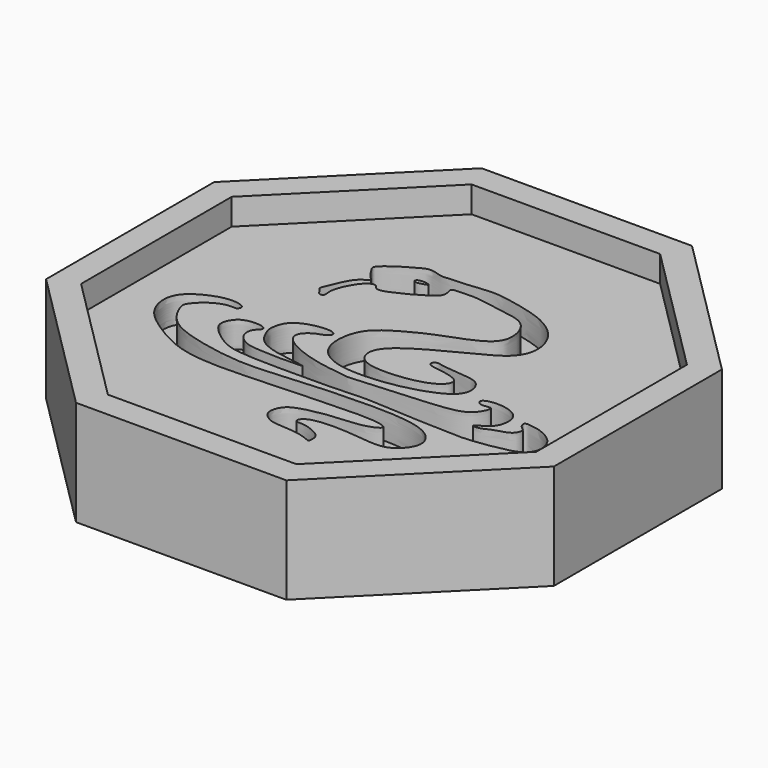
from build123d import *

# Parameters (mm, degrees)
F1_DEPTH = 25.4
F3_DEPTH = 6.35
F5_DEPTH = 6.35


with BuildPart() as f1:
    # F0 (on Top) → F1 (new body)
    with BuildSketch(Plane.XY):
        Polygon((-61.3372846899, 25.3607087968), (-61.3047391097, -25.4392807779), (-25.3607087968, -61.3372846899), (25.4392807779, -61.3047391097), (61.3372846899, -25.3607087968), (61.3047391097, 25.4392807779), (25.3607087968, 61.3372846899), (-25.4392807779, 61.3047391097), align=None)
    extrude(amount=F1_DEPTH)

    # F2 (on face) → F3 (cut)
    with BuildSketch(Plane.XY.offset(25.4)):
        Polygon((-54.9856008905, 22.734521413), (-54.9564255154, -22.8049569991), (-22.734521413, -54.9856008905), (22.8049569991, -54.9564255154), (54.9856008905, -22.734521413), (54.9564255154, 22.8049569991), (22.734521413, 54.9856008905), (-22.8049569991, 54.9564255154), align=None)
    extrude(amount=-F3_DEPTH, mode=Mode.SUBTRACT)

    # F4 (on face) → F5 (cut)
    with BuildSketch(Plane.XY.offset(19.05)):
        with BuildLine():
            add(Edge.make_bspline(
                [(0, 32.4928350747), (-2.02665443, 32.4515584663), (-6.1821896181, 31.7497065716), (-9.3396897547, 31.9242783794), (-11.5003480916, 31.3913149272), (-14.4774634916, 32.8444451189), (-17.4734169272, 31.4267092211), (-24.3950179391, 27.1323443805), (-23.4189738768, 25.4150859361), (-21.7980747865, 22.8958449868), (-20.2814454001, 21.9562019156), (-23.4921452503, 21.1361770855), (-25.5825772036, 15.5301374946), (-26.6320070635, 13.378526896), (-25.6067459699, 12.798784515), (-25.1286460968, 11.4356624756), (-23.5210478416, 11.6468537322), (-24.6057192979, 14.0162008911), (-21.7647301762, 20.1265801161), (-18.9984353167, 21.4468623697), (-18.2021783197, 20.2606055269), (-16.9086613099, 19.2202016185), (-8.4702710322, 23.5975113963), (-5.6737203544, 26.0508520587), (-7.1692394224, 28.9077254429), (-4.1932743401, 28.6342846216), (-1.3567965699, 29.1457740371), (6.2167864003, 27.5901948262), (12.9549170867, 26.8400806968), (15.0609285948, 20.5636192608), (13.0100880074, 15.7885773924), (2.3628006843, 12.4674207824), (-4.7571848216, 8.6961838701), (-10.0291084028, 4.8197671989), (-11.1670998303, -3.5430268416), (-6.7071414645, -8.6049913594), (2.3622730255, -9.7875455052), (14.1658166841, -8.0563944992), (22.8447425092, -3.8696651926), (21.7660557386, 1.3325554585), (18.9384588869, 2.8112387978), (11.9729408281, 2.9638757064), (10.5506555229, 3.6067465992), (9.3420681736, 3.362953775), (9.0839535739, 1.8237552438), (12.1699293236, 1.6448938693), (17.3275762328, 0.5228914679), (17.343957002, -1.7418792899), (14.2201592243, -4.5982214393), (3.8219661075, -6.0350042747), (-1.8054793689, -4.5760486927), (-3.159852163, -0.998458362), (-1.1271792202, 2.8134408354), (6.1106781025, 7.1885070336), (13.2013933579, 10.8338087429), (19.383236378, 13.9073936379), (22.0141910817, 18.6787142044), (20.5131648158, 24.9752478489), (14.6555355139, 29.917176979), (5.4072057042, 31.8795066229), (1.8888431912, 32.5313048994), (0, 32.4928350747)],
                knots=[0, 0, 0, 0, 0.0206390772, 0.0351612434, 0.0470236164, 0.0609195804, 0.0763934194, 0.0988147036, 0.1085593451, 0.1231309925, 0.131614117, 0.1439249136, 0.1644005417, 0.1761612399, 0.1839691152, 0.1934029176, 0.2013357647, 0.2128550407, 0.2341653825, 0.2471110948, 0.2555942041, 0.2647630615, 0.2897604539, 0.3052972595, 0.3168235043, 0.3283890295, 0.3428366407, 0.36564551, 0.3865657196, 0.4057498968, 0.4231186957, 0.4500471985, 0.4739033938, 0.4942297055, 0.5166925362, 0.5365755735, 0.5607938567, 0.5899783508, 0.6138798307, 0.6299465505, 0.644394163, 0.6658774806, 0.6761912827, 0.684313521, 0.6922489115, 0.7059324809, 0.7244501375, 0.7343952618, 0.750269063, 0.7770640906, 0.7962909332, 0.8105296101, 0.8265963281, 0.8503692785, 0.8741628976, 0.8953677377, 0.9135255692, 0.9333499073, 0.9557795967, 0.9807643672, 1, 1, 1, 1], degree=3))
        make_face()
        with BuildLine():
            add(Edge.make_bspline(
                [(-11.1860819161, 27.4196639657), (-11.2563861036, 27.6936958998), (-14.0012109775, 28.0926169968), (-14.4442728998, 26.7279262694), (-13.140761497, 26.6447598295), (-12.6349676031, 26.846565007), (-11.1346868455, 27.2193360607), (-11.1860819161, 27.4196639657)],
                knots=[0, 0, 0, 0, 0.2889826517, 0.4525434925, 0.6261316853, 0.7887425441, 1, 1, 1, 1], degree=3))
        make_face(mode=Mode.SUBTRACT)
        with BuildLine():
            add(Edge.make_bspline(
                [(-1.1664102785, -11.3425226882), (-2.4842779162, -11.1486337497), (-8.5526134999, -10.5839010924), (-17.4794108044, -7.0572240397), (-18.266327002, -3.4826760224), (-15.5125530603, -1.4249147337), (-13.9166212665, -1.1184361923), (-12.3717590035, -0.1211327365), (-12.9132368388, 1.3984629466), (-18.0138444325, 1.2150440539), (-22.723019617, -1.0848573406), (-23.3972945312, -4.862435008), (-23.2066140331, -6.319579442), (-21.213254088, -11.1518322288), (-13.9789421106, -12.5984399396), (-6.9455404486, -13.4703228485), (-13.8877543431, -13.5975285068), (-19.1807216844, -13.4215999201), (-23.1423440865, -13.0469543081), (-26.0361310429, -10.5001925504), (-25.805753022, -7.5652206626), (-23.8512704233, -6.3589419892), (-25.1921291192, -5.0510765266), (-29.8789552059, -5.219172169), (-31.7129141235, -7.769440464), (-32.4023710313, -10.7210577986), (-26.2596721529, -15.5877879415), (-21.6584048851, -16.5387829646), (-14.4649421135, -16.836098081), (-4.9521619341, -16.7420522294), (1.6190281119, -16.7650158379), (8.3152182991, -16.1939516039), (15.5185187492, -16.7765146578), (20.308012588, -17.0719490808), (25.998198314, -17.1662026151), (33.1690536304, -17.6579269433), (39.6248516906, -16.6685545513), (46.0747675359, -15.4046066885), (47.7530334862, -11.9241209977), (46.6328452738, -7.9311136006), (42.4461470585, -5.8555307024), (40.6548102856, -5.6076176981), (38.1970955586, -5.1724477526), (38.4025358872, -6.6053706812), (39.2974932883, -7.4005381024), (40.1235339059, -7.9631310224), (39.5173708689, -9.7522862567), (37.809112654, -10.7285822467), (34.7975424818, -11.3939970567), (33.3296774157, -12.4661493109), (30.4251730138, -12.6112461847), (33.721203786, -10.7900236231), (35.3440376001, -9.193064247), (35.8460607238, -5.4109887905), (33.3830752712, -2.7753889232), (28.2549505247, -2.216551509), (25.6219858577, -3.4403034809), (27.1148180657, -5.1379482274), (30.2034505279, -3.9464711824), (29.0055185388, -7.0257362536), (26.217286788, -9.9832002985), (14.1105261465, -10.4663841793), (2.3695856708, -11.5838239957), (0.0200399681, -11.5738681482), (-0.6349572405, -11.4207117737), (-1.1664102785, -11.3425226882)],
                knots=[0, 0, 0, 0, 0.0223691706, 0.0480568622, 0.0615710219, 0.0759244025, 0.0869793068, 0.0972682223, 0.1053337035, 0.1232981087, 0.1423408108, 0.1573783055, 0.1674794599, 0.1849112758, 0.20845467, 0.225461068, 0.2423440146, 0.2629390182, 0.2791973751, 0.2945983023, 0.307926129, 0.318951274, 0.3279256957, 0.3453707221, 0.3595622846, 0.3726377905, 0.3947448203, 0.4130857268, 0.4351742017, 0.4609506109, 0.4822965348, 0.5037982154, 0.526029278, 0.5441840249, 0.5638361393, 0.5860562606, 0.607775166, 0.6283736085, 0.6433309743, 0.6594596769, 0.6767363495, 0.6886846896, 0.7002122469, 0.7081670213, 0.7173937428, 0.7250317942, 0.7353310189, 0.7470311187, 0.7613878839, 0.773411782, 0.7837835217, 0.7967086809, 0.8100953088, 0.8252145642, 0.8401779107, 0.8590754412, 0.8710935792, 0.8810151755, 0.8935927763, 0.9052803493, 0.9214090515, 0.9505372178, 0.9793705096, 0.990979243, 1, 1, 1, 1], degree=3))
        make_face()
        with BuildLine():
            add(Edge.make_bspline(
                [(-41.9709534322, -9.0136790223), (-42.1911620114, -8.3583932618), (-42.34969998, -7.2405928655), (-38.6528197879, -3.4410600635), (-34.7540509361, -2.5842009589), (-33.473796151, -2.9777589907), (-32.8485086334, -2.1837376094), (-32.9772793951, -1.1963546931), (-36.114841486, -0.5046797806), (-40.0271404038, -1.3424478879), (-44.9068911973, -3.8909175217), (-46.9786196208, -7.8426469478), (-45.4738964104, -13.7069461942), (-39.4481143266, -18.2535337581), (-29.8342522455, -23.8493289435), (-12.6099116362, -23.2191159228), (3.9874574831, -22.4000367715), (15.7226173903, -22.0578064491), (19.6371595731, -23.462862165), (15.1348280873, -25.5917400241), (9.3340607209, -25.5872860996), (1.4238978196, -26.9538303197), (-1.799372016, -28.7679988153), (-2.7785407451, -32.688769696), (0.0580706355, -34.5161638938), (1.5270121873, -34.9655891739), (6.7559561268, -35.0964780058), (9.951827923, -36.0602842107), (11.0358232658, -36.7719422221), (11.2336976109, -35.2179528538), (10.6711227715, -33.3342328553), (6.2510157141, -31.599622017), (3.6434816701, -32.0568229039), (4.6599594673, -29.0922304053), (13.4006095047, -28.8309592901), (19.622244979, -29.7672833203), (25.1671195784, -29.9594311524), (29.7281007289, -24.4418042796), (25.2842929097, -18.0860589173), (8.9325042094, -17.8795427516), (-4.5802673011, -18.4493811924), (-17.6398430541, -19.9798226398), (-29.383236807, -18.1262721061), (-39.2922691717, -15.0747253717), (-41.5602476096, -10.2358370249), (-41.9709534322, -9.0136790223)],
                knots=[0, 0, 0, 0, 0.0132399726, 0.0362285429, 0.0568027573, 0.0677544837, 0.0769773246, 0.0856997561, 0.102886405, 0.1241131012, 0.1479141258, 0.1687284592, 0.1926640754, 0.2204788884, 0.2542958038, 0.2968377572, 0.3402436916, 0.3755917119, 0.3909335712, 0.4095268725, 0.4358957765, 0.4649601583, 0.48429607, 0.5030039239, 0.5203658503, 0.5335172464, 0.5570313887, 0.5763929492, 0.5856565788, 0.5965049086, 0.6105986869, 0.6329057833, 0.6473315524, 0.6604771391, 0.6901223856, 0.7172238816, 0.7406004101, 0.7651963995, 0.7897320009, 0.8306224765, 0.8697409284, 0.9067128362, 0.9425691187, 0.9753064396, 1, 1, 1, 1], degree=3))
        make_face()
    extrude(amount=-F5_DEPTH, mode=Mode.SUBTRACT)


solid = f1.part
